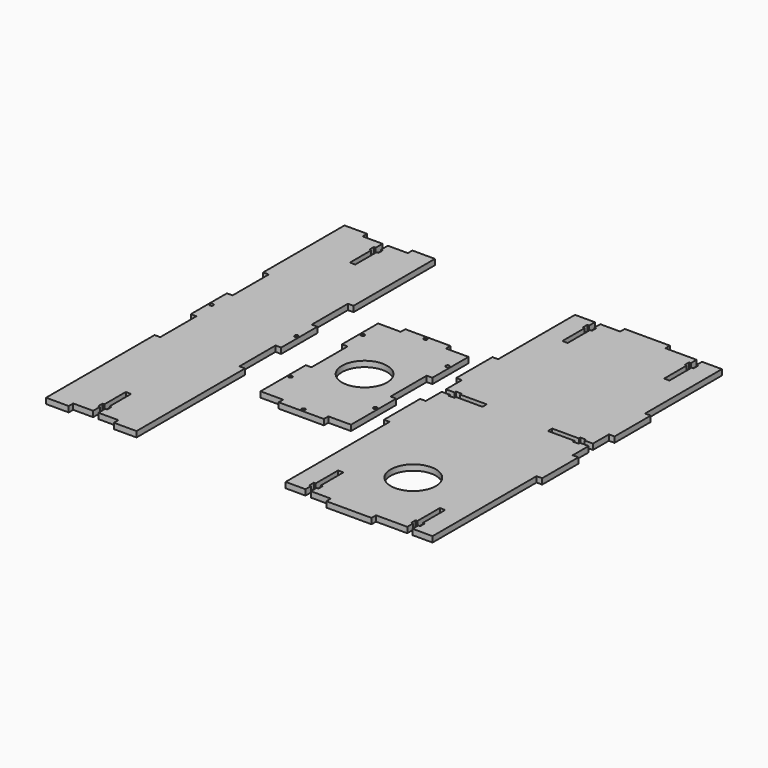
from build123d import *

# Parameters (mm, degrees)
F0_R     = 1
F0_R_2   = 12.7
F2_DEPTH = 3.175
F1_R     = 1
F3_DEPTH = 3.175
F4_R     = 12.7
F4_W     = 25.4
F4_H     = 3.175
F5_DEPTH = 3.175


# Not quite as in the source:
# - a length typed as a fraction of an inch, garbled in the dataset ("3 / 203.2 mm" for 3/8 in), is restored


with BuildPart() as f2:
    # F0 (on Top) → F2 (new body)
    with BuildSketch(Plane.XY):
        Polygon((-12.7, 41.275), (-22.225, 41.275), (-25.4, 41.275), (-25.4, 15.875), (-22.225, 15.875), (-22.225, -9.525), (-25.4, -9.525), (-25.4, -34.925), (-25.4, -41.275), (-22.225, -41.275), (-12.7, -41.275), (-12.7, -44.45), (12.7, -44.45), (12.7, -41.275), (22.225, -41.275), (25.4, -41.275), (25.4, -34.925), (25.4, -9.525), (22.225, -9.525), (22.225, 15.875), (25.4, 15.875), (25.4, 41.275), (22.225, 41.275), (12.7, 41.275), (12.7, 44.45), (-12.7, 44.45), align=None)
        with Locations((0, -42.8625)):
            Circle(F0_R, mode=Mode.SUBTRACT)
        with Locations((-23.8125, -22.225)):
            Circle(F0_R, mode=Mode.SUBTRACT)
        with Locations((23.8125, -22.225)):
            Circle(F0_R, mode=Mode.SUBTRACT)
        Circle(F0_R_2, mode=Mode.SUBTRACT)
        with Locations((-23.8125, 28.575)):
            Circle(F0_R, mode=Mode.SUBTRACT)
        with Locations((0, 42.8625)):
            Circle(F0_R, mode=Mode.SUBTRACT)
        with Locations((23.8125, 28.575)):
            Circle(F0_R, mode=Mode.SUBTRACT)
    extrude(amount=F2_DEPTH)


with BuildPart() as f3:
    # F1 (on Top) → F3 (new body)
    with BuildSketch(Plane.XY):
        Polygon((-71.1853192556, 101.6), (-82.385493889, 101.6), (-82.385493889, 104.775), (-95.085493889, 104.775), (-95.085493889, 101.6), (-95.085493889, 47.625), (-91.910493889, 47.625), (-91.910493889, 22.225), (-95.085493889, 22.225), (-95.085493889, -3.175), (-91.910493889, -3.175), (-91.910493889, -28.575), (-95.085493889, -28.575), (-95.085493889, -101.6), (-95.085493889, -104.775), (-82.385493889, -104.775), (-82.385493889, -101.6), (-71.1853192556, -101.6), (-71.1853192556, -96.8375), (-72.225493889, -96.8375), (-72.225493889, -93.6625), (-71.1853192556, -93.6625), (-71.1853192556, -78.6942235994), (-68.1856685224, -78.74), (-68.1856685224, -93.6625), (-67.145493889, -93.6625), (-67.145493889, -96.8375), (-68.1856685224, -96.8375), (-68.1856685224, -101.6), (-56.985493889, -101.6), (-56.985493889, -104.775), (-44.285493889, -104.775), (-44.285493889, -101.6), (-44.285493889, -28.575), (-47.460493889, -28.575), (-47.460493889, -3.175), (-44.285493889, -3.175), (-44.285493889, 22.225), (-47.460493889, 22.225), (-47.460493889, 47.625), (-44.285493889, 47.625), (-44.285493889, 101.6), (-44.285493889, 104.775), (-56.985493889, 104.775), (-56.985493889, 101.6), (-68.1856685224, 101.6), (-68.1856685224, 96.8375), (-67.145493889, 96.8375), (-67.145493889, 93.6625), (-68.1856685224, 93.6625), (-68.1856685224, 78.74), (-71.1853192556, 78.6942235994), (-71.1853192556, 93.6625), (-72.225493889, 93.6625), (-72.225493889, 96.8375), (-71.1853192556, 96.8375), align=None)
        with Locations((-93.497993889, 9.525)):
            Circle(F1_R, mode=Mode.SUBTRACT)
        with Locations((-45.872993889, 9.525)):
            Circle(F1_R, mode=Mode.SUBTRACT)
    extrude(amount=F3_DEPTH)


with BuildPart() as f5:
    # F4 (on Top) → F5 (new body)
    with BuildSketch(Plane.XY):
        Polygon((48.1215686488, 101.6), (36.9215686488, 101.6), (36.9215686488, 47.625), (33.7465686488, 47.625), (33.7465686488, 22.225), (36.9215686488, 22.225), (36.9215686488, 11.0249418534), (41.6840686488, 11.0249418534), (41.6840686488, 12.065), (44.8590686488, 12.065), (44.8590686488, 11.0249418534), (59.7815686488, 11.0249418534), (59.8079835334, 8.0250581466), (44.8590686488, 8.0250581466), (44.8590686488, 6.985), (41.6840686488, 6.985), (41.6840686488, 8.0250581466), (36.9215686488, 8.0250581466), (36.9215686488, -3.175), (33.7465686488, -3.175), (33.7465686488, -28.575), (36.9215686488, -28.575), (36.9215686488, -101.6), (48.1215686488, -101.6), (48.1215686488, -97.6185846567), (47.0815686488, -97.6185846567), (47.0815686488, -94.4435846567), (48.1215686488, -94.4435846567), (48.1215686488, -78.74), (51.1215686488, -78.74), (51.1215686488, -94.4435846567), (52.1615686488, -94.4435846567), (52.1615686488, -97.6185846567), (51.1215686488, -97.6185846567), (51.1215686488, -101.6), (62.3215686488, -101.6), (87.7215686488, -101.6), (105.2715686488, -101.6), (105.2715686488, -97.6185846567), (104.2315686488, -97.6185846567), (104.2315686488, -94.4435846567), (105.2715686488, -94.4435846567), (105.2715686488, -78.74), (108.2715686488, -78.74), (108.2715686488, -94.4435846567), (109.3115686488, -94.4435846567), (109.3115686488, -97.6185846567), (108.2715686488, -97.6185846567), (108.2715686488, -101.6), (119.4715686488, -101.6), (119.4715686488, -28.575), (122.6465686488, -28.575), (122.6465686488, -3.175), (119.4715686488, -3.175), (119.4715686488, 8.0250581466), (114.7090686488, 8.0250581466), (114.7090686488, 6.985), (111.5340686488, 6.985), (111.5340686488, 8.0250581466), (96.585153764, 8.0250581466), (96.6115686488, 11.0249418534), (111.5340686488, 11.0249418534), (111.5340686488, 12.065), (114.7090686488, 12.065), (114.7090686488, 11.0249418534), (119.4715686488, 11.0249418534), (119.4715686488, 22.225), (122.6465686488, 22.225), (122.6465686488, 47.625), (119.4715686488, 47.625), (119.4715686488, 101.6), (108.2715686488, 101.6), (108.2715686488, 97.6185846567), (109.3115686488, 97.6185846567), (109.3115686488, 94.4435846567), (108.2715686488, 94.4435846567), (108.2715686488, 78.74), (105.2715686488, 78.74), (105.2715686488, 94.4435846567), (104.2315686488, 94.4435846567), (104.2315686488, 97.6185846567), (105.2715686488, 97.6185846567), (105.2715686488, 101.6), (87.7215686488, 101.6), (62.3215686488, 101.6), (51.1215686488, 101.6), (51.1215686488, 97.6185846567), (52.1615686488, 97.6185846567), (52.1615686488, 94.4435846567), (51.1215686488, 94.4435846567), (51.1215686488, 78.74), (48.1215686488, 78.74), (48.1215686488, 94.4435846567), (47.0815686488, 94.4435846567), (47.0815686488, 97.6185846567), (48.1215686488, 97.6185846567), align=None)
        with Locations((78.1965686488, -63.5)):
            Circle(F4_R, mode=Mode.SUBTRACT)
        with Locations((75.0215686488, -103.1875)):
            Rectangle(F4_W, F4_H)
        with Locations((75.0215686488, 103.1875)):
            Rectangle(F4_W, F4_H)
    extrude(amount=F5_DEPTH)


solid = Compound([f2.part, f3.part, f5.part])
